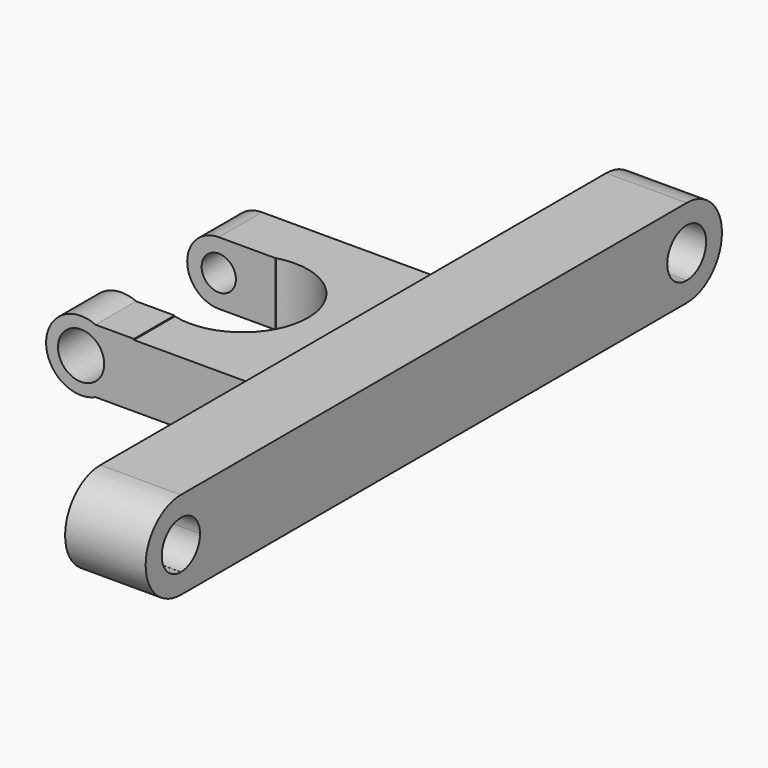
from build123d import *

# Parameters (mm, degrees)
F1_DEPTH = 25.4
F3_DEPTH = 9.906
F4_R     = 5.4054687582
F5_DEPTH = 17.018
F7_DEPTH = 16.002


# Not quite as in the source:
# - ends of sketch curves that miss each other by under 0.0002 mm in the source are joined


with BuildPart() as f1:
    # F0 (on Right) → F1 (new body)
    with BuildSketch(Plane.YZ):
        with BuildLine():
            Line((-99.6930599213, 7.5515317731), (-99.6930599213, 13.8873864871))
            ThreePointArc((-99.6930599213, 13.8873864871), (-113.5804464084, 0), (-99.6930599213, -13.8873864871))
            Line((-99.6930599213, -13.8873864871), (-99.6930599213, -7.5509602816))
            ThreePointArc((-99.6930599213, -7.5509602816), (-104.2631477896, -6.0002098207), (-106.9606792933, -1.9984784576))
            ThreePointArc((-106.9606792933, -1.9984784576), (-107.2304460851, -0.0041593028), (-106.9628804792, 1.9904563644))
            ThreePointArc((-106.9628804792, 1.9904563644), (-104.2749842635, 5.9848237142), (-99.7176355394, 7.5373431398))
            ThreePointArc((-99.7176355394, 7.5373431398), (-99.7053477533, 7.5373772953), (-99.6930599213, 7.5373873115))
            Line((-99.6930599213, 7.5373873115), (-99.6930599213, 7.5515317731))
        make_face()
        with BuildLine():
            Line((99.6930599213, 13.8873864871), (-99.6930599213, 13.8873864871))
            Line((-99.6930599213, 13.8873864871), (-99.6930599213, 7.5515317731))
            ThreePointArc((-99.6930599213, 7.5515317731), (-94.3533205962, 5.3397393251), (-92.1415281482, 0))
            ThreePointArc((-92.1415281482, 0), (-94.3541776231, -5.33475565), (-99.6930599995, -7.5374291426))
            Line((-99.6930599995, -7.5374291426), (-99.6930599213, -7.5509602816))
            Line((-99.6930599213, -7.5509602816), (-99.6930599213, -13.8873864871))
            Line((-99.6930599213, -13.8873864871), (99.6930599213, -13.8873864871))
            Line((99.6930599213, -13.8873864871), (99.6930599213, -7.671022612))
            ThreePointArc((99.6930599213, -7.671022612), (94.2688278137, -5.4242321076), (92.0220373093, 0))
            ThreePointArc((92.0220373093, 0), (92.1497116605, 1.39373058), (92.5284847617, 2.7410674375))
            ThreePointArc((92.5284847617, 2.7410674375), (95.3446235575, 6.3194690523), (99.6930599213, 7.671022612))
            Line((99.6930599213, 7.671022612), (99.6930599213, 13.8873864871))
        make_face()
        with BuildLine():
            ThreePointArc((99.6930599213, -13.8873864871), (113.5804464084, 0), (99.6930599213, 13.8873864871))
            Line((99.6930599213, 13.8873864871), (99.6930599213, 7.671022612))
            ThreePointArc((99.6930599213, 7.671022612), (107.3640825332, 0), (99.6930599213, -7.671022612))
            Line((99.6930599213, -7.671022612), (99.6930599213, -13.8873864871))
        make_face()
    extrude(amount=F1_DEPTH)

    # F2 (on Top) → F3 (join, symmetric)
    with BuildSketch(Plane.XY):
        with BuildLine():
            Line((0, 0), (0, 36.4271812141))
            Line((0, 36.4271812141), (-39.9832986295, 36.4271812141))
            Line((-39.9832986295, 36.4271812141), (-39.9832986295, 19.475013286))
            ThreePointArc((-39.9832986295, 19.475013286), (-13.9090954175, -0.413186714), (-39.9832986295, -20.301386714))
            Line((-39.9832986295, -20.301386714), (-39.9832986295, -36.4658497274))
            Line((-39.9832986295, -36.4658497274), (0, -36.4658497274))
            Line((0, -36.4658497274), (0, -36.4271812141))
            Line((0, -36.4271812141), (0, 0))
        make_face()
    extrude(amount=F3_DEPTH, both=True)

    # F4 (on face) → F5 (join)
    with BuildSketch(Plane(origin=(0, 36.4271812141, 0), x_dir=(-1, 0, 0), z_dir=(0, 1, 0))):
        with BuildLine():
            Line((57.9356960952, 9.906), (39.9832986295, 9.906))
            Line((39.9832986295, 9.906), (39.9832986295, -9.906))
            Line((39.9832986295, -9.906), (39.9832986295, -9.9966842681))
            Line((39.9832986295, -9.9966842681), (57.9356960952, -9.9966842681))
            ThreePointArc((57.9356960952, -9.9966842681), (67.8870382293, -0.0453421341), (57.9356960952, 9.906))
        make_face()
        with Locations((57.9356960952, -0.0453421341)):
            Circle(F4_R, mode=Mode.SUBTRACT)
    extrude(amount=-F5_DEPTH)

    # F6 (on face) → F7 (join)
    with BuildSketch(Plane.XZ.offset(36.4658497274)):
        with BuildLine():
            Line((-52.1078817546, -9.906), (-39.9832986295, -9.906))
            Line((-39.9832986295, -9.906), (-39.9832986295, 9.906))
            Line((-39.9832986295, 9.906), (-39.9832986295, 10.2091357112))
            Line((-39.9832986295, 10.2091357112), (-52.1078817546, 10.2091357112))
            Line((-52.1078817546, 10.2091357112), (-52.1078817546, 5.8468863204))
            ThreePointArc((-52.1078817546, 5.8468863204), (-50.0877827712, 3.3118599928), (-49.366872241, 0.1515678556))
            ThreePointArc((-49.366872241, 0.1515678556), (-50.0877827712, -3.0087242816), (-52.1078817546, -5.5437506092))
            Line((-52.1078817546, -5.5437506092), (-52.1078817546, -9.906))
        make_face()
        with BuildLine():
            ThreePointArc((-52.1078817546, 10.2091357112), (-67.6917094663, 0.1515678556), (-52.1078817546, -9.906))
            Line((-52.1078817546, -9.906), (-52.1078817546, -5.5437506092))
            ThreePointArc((-52.1078817546, -5.5437506092), (-63.9417160607, 0.1515678556), (-52.1078817546, 5.8468863204))
            Line((-52.1078817546, 5.8468863204), (-52.1078817546, 10.2091357112))
        make_face()
    extrude(amount=-F7_DEPTH)


solid = f1.part
